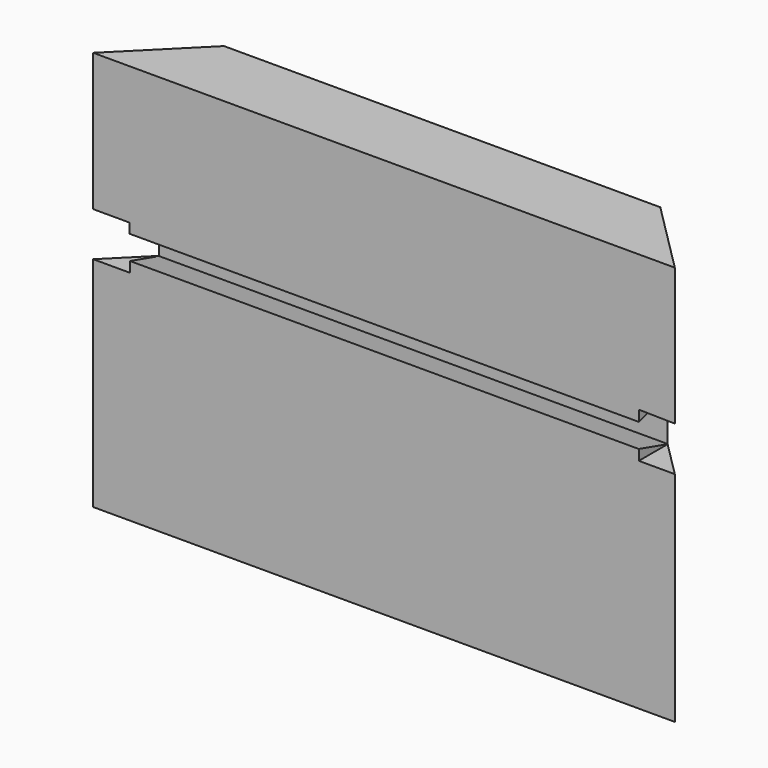
from build123d import *

# Parameters (mm, degrees)
F1_DEPTH  = 6.35
F3_DEPTH  = 279.4
F4_W      = 101.6
F4_H      = 3.175
F5_DEPTH  = 3.175
F6_W      = 12.7
F6_H      = 4.1792877018
F7_DEPTH  = 25.4
F8_W      = 101.6
F8_H      = 6.35
F9_DEPTH  = 25.4
F11_DEPTH = 69.851
F12_W     = 6.2937450767
F12_H     = 5.9905603992
F13_DEPTH = 6.35
F14_W     = 6.4354827628
F14_H     = 1.8108228737
F15_DEPTH = 25.4
F16_W     = 6.3454108313
F16_H     = 1.71593274
F17_DEPTH = 25.4


# Not quite as in the source:
# - a feature names something its author has since deleted; it is built from what else it names


with BuildPart() as f1:
    # F0 (on Front) → F1 (new body, symmetric)
    with BuildSketch(Plane.XZ):
        Polygon((0, 38.1), (0, 0), (101.6, 0), (101.6, 76.2), (0, 76.2), align=None)
    extrude(amount=F1_DEPTH, both=True)

    # F2 (on face) → F3 (cut)
    with BuildSketch(Plane(origin=(0, 0, 0), x_dir=(0, -1, 0), z_dir=(-1, 0, 0))):
        Polygon((0, 45.9105), (0, 38.1), (6.35, 39.9208331996), (6.35, 44.0896668004), align=None)
    extrude(amount=-F3_DEPTH, mode=Mode.SUBTRACT)

    # F4 (on face) → F5 (cut)
    with BuildSketch(Plane(origin=(0, 6.35, 0), x_dir=(-1, 0, 0), z_dir=(0, 1, 0))):
        with Locations((-50.8, 4.7625)):
            Rectangle(F4_W, F4_H)
    extrude(amount=-F5_DEPTH, mode=Mode.SUBTRACT)

    # F6 (on face) → F7 (cut)
    with BuildSketch(Plane.XZ):
        with BuildLine():
            Line((50.8, 39.8820452392), (50.8, 44.0613329411))
            ThreePointArc((50.8, 44.0613329411), (48.7103561491, 41.9716890901), (50.8, 39.8820452392))
        make_face()
        with Locations((57.15, 41.9716890901)):
            Rectangle(F6_W, F6_H)
        with BuildLine():
            ThreePointArc((63.5, 39.8820452392), (65.5896438509, 41.9716890901), (63.5, 44.0613329411))
            Line((63.5, 44.0613329411), (63.5, 39.8820452392))
        make_face()
    extrude(amount=-F7_DEPTH, mode=Mode.SUBTRACT)

    # F8 (on face) → F9 (cut)
    with BuildSketch(Plane.XZ.offset(6.35)):
        with Locations((50.8, 73.025)):
            Rectangle(F8_W, F8_H)
    extrude(amount=-F9_DEPTH, mode=Mode.SUBTRACT)

    # F10 (on face) → F11 (cut, through all)
    with BuildSketch(Plane.XY.offset(69.85)):
        Polygon((0, 6.35), (0, -6.35), (12.7, 6.35), align=None)
        Polygon((88.9, 6.35), (101.6, -6.35), (101.6, 6.35), align=None)
    extrude(amount=-F11_DEPTH, mode=Mode.SUBTRACT)

    # F12 (on face) → F13 (cut)
    with BuildSketch(Plane.XZ.offset(6.35)):
        with Locations((98.4531274617, 41.0943866008)):
            Rectangle(F12_W, F12_H)
        Polygon((101.6, 45.8681471646), (95.3062549233, 45.9736101329), (95.3062549233, 44.0896668004), (101.6, 44.0896668004), align=None)
    extrude(amount=-F13_DEPTH, mode=Mode.SUBTRACT)

    # F14 (on face) → F15 (cut)
    with BuildSketch(Plane.XZ.offset(6.35)):
        with Locations((3.2177413814, 39.0154217627)):
            Rectangle(F14_W, F14_H)
    extrude(amount=-F15_DEPTH, mode=Mode.SUBTRACT)

    # F16 (on face) → F17 (cut)
    with BuildSketch(Plane.XZ.offset(6.35)):
        with Locations((3.1727054156, 44.9476331705)):
            Rectangle(F16_W, F16_H)
    extrude(amount=-F17_DEPTH, mode=Mode.SUBTRACT)


solid = f1.part
